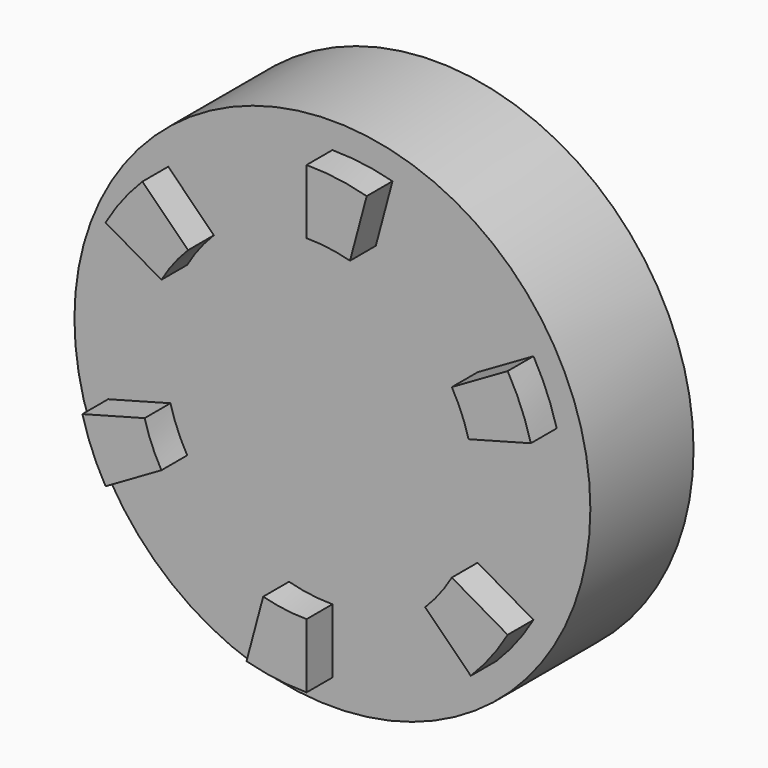
from build123d import *

# Parameters (mm, degrees)
F0_R     = 25.4
F1_DEPTH = 12.7
F2_DEPTH = 15.875


# Not quite as in the source:
# - a length typed as a fraction of an inch, garbled in the dataset ("3 / 203.2 mm" for 3/8 in), is restored
# - a feature names something its author has since deleted; it is built from what else it names


with BuildPart() as f1:
    # F0 (on Front) → F1 (new body)
    with BuildSketch(Plane.XZ):
        Circle(F0_R)
        with BuildLine():
            Line((0, -16.51), (0, -22.86))
            ThreePointArc((0, -22.86), (-2.9838287542, -22.664429531), (-5.916603371, -22.081064389))
            Line((-5.916603371, -22.081064389), (-4.2731024346, -15.947435392))
            ThreePointArc((-4.2731024346, -15.947435392), (-2.1549874336, -16.3687546613), (0, -16.51))
        make_face(mode=Mode.SUBTRACT)
        with BuildLine():
            Line((-14.2980794165, -8.255), (-19.7973407305, -11.43))
            ThreePointArc((-19.7973407305, -11.43), (-21.1198861132, -8.7481432639), (-22.081064389, -5.916603371))
            Line((-22.081064389, -5.916603371), (-15.947435392, -4.2731024346))
            ThreePointArc((-15.947435392, -4.2731024346), (-15.2532510818, -6.3181034683), (-14.2980794165, -8.255))
        make_face(mode=Mode.SUBTRACT)
        with BuildLine():
            Line((14.2980794165, -8.255), (19.7973407305, -11.43))
            ThreePointArc((19.7973407305, -11.43), (18.1360573591, -13.9162862671), (16.1644610179, -16.1644610179))
            Line((16.1644610179, -16.1644610179), (11.6743329574, -11.6743329574))
            ThreePointArc((11.6743329574, -11.6743329574), (13.0982636482, -10.0506511929), (14.2980794165, -8.255))
        make_face(mode=Mode.SUBTRACT)
        with BuildLine():
            Line((-14.2980794165, 8.255), (-19.7973407305, 11.43))
            ThreePointArc((-19.7973407305, 11.43), (-18.1360573591, 13.9162862671), (-16.1644610179, 16.1644610179))
            Line((-16.1644610179, 16.1644610179), (-11.6743329574, 11.6743329574))
            ThreePointArc((-11.6743329574, 11.6743329574), (-13.0982636482, 10.0506511929), (-14.2980794165, 8.255))
        make_face(mode=Mode.SUBTRACT)
        with BuildLine():
            Line((14.2980794165, 8.255), (19.7973407305, 11.43))
            ThreePointArc((19.7973407305, 11.43), (21.1198861132, 8.7481432639), (22.081064389, 5.916603371))
            Line((22.081064389, 5.916603371), (15.947435392, 4.2731024346))
            ThreePointArc((15.947435392, 4.2731024346), (15.2532510818, 6.3181034683), (14.2980794165, 8.255))
        make_face(mode=Mode.SUBTRACT)
        with BuildLine():
            Line((0, 16.51), (0, 22.86))
            ThreePointArc((0, 22.86), (2.9838287542, 22.664429531), (5.916603371, 22.081064389))
            Line((5.916603371, 22.081064389), (4.2731024346, 15.947435392))
            ThreePointArc((4.2731024346, 15.947435392), (2.1549874336, 16.3687546613), (0, 16.51))
        make_face(mode=Mode.SUBTRACT)
        with BuildLine():
            ThreePointArc((5.916603371, 22.081064389), (2.9838287542, 22.664429531), (0, 22.86))
            Line((0, 22.86), (0, 16.51))
            ThreePointArc((0, 16.51), (2.1549874336, 16.3687546613), (4.2731024346, 15.947435392))
            Line((4.2731024346, 15.947435392), (5.916603371, 22.081064389))
        make_face()
        with BuildLine():
            ThreePointArc((-16.1644610179, 16.1644610179), (-18.1360573591, 13.9162862671), (-19.7973407305, 11.43))
            Line((-19.7973407305, 11.43), (-14.2980794165, 8.255))
            ThreePointArc((-14.2980794165, 8.255), (-13.0982636482, 10.0506511929), (-11.6743329574, 11.6743329574))
            Line((-11.6743329574, 11.6743329574), (-16.1644610179, 16.1644610179))
        make_face()
        with BuildLine():
            ThreePointArc((-22.081064389, -5.916603371), (-21.1198861132, -8.7481432639), (-19.7973407305, -11.43))
            Line((-19.7973407305, -11.43), (-14.2980794165, -8.255))
            ThreePointArc((-14.2980794165, -8.255), (-15.2532510818, -6.3181034683), (-15.947435392, -4.2731024346))
            Line((-15.947435392, -4.2731024346), (-22.081064389, -5.916603371))
        make_face()
        with BuildLine():
            ThreePointArc((16.1644610179, -16.1644610179), (18.1360573591, -13.9162862671), (19.7973407305, -11.43))
            Line((19.7973407305, -11.43), (14.2980794165, -8.255))
            ThreePointArc((14.2980794165, -8.255), (13.0982636482, -10.0506511929), (11.6743329574, -11.6743329574))
            Line((11.6743329574, -11.6743329574), (16.1644610179, -16.1644610179))
        make_face()
        with BuildLine():
            ThreePointArc((22.081064389, 5.916603371), (21.1198861132, 8.7481432639), (19.7973407305, 11.43))
            Line((19.7973407305, 11.43), (14.2980794165, 8.255))
            ThreePointArc((14.2980794165, 8.255), (15.2532510818, 6.3181034683), (15.947435392, 4.2731024346))
            Line((15.947435392, 4.2731024346), (22.081064389, 5.916603371))
        make_face()
        with BuildLine():
            ThreePointArc((-5.916603371, -22.081064389), (-2.9838287542, -22.664429531), (0, -22.86))
            Line((0, -22.86), (0, -16.51))
            ThreePointArc((0, -16.51), (-2.1549874336, -16.3687546613), (-4.2731024346, -15.947435392))
            Line((-4.2731024346, -15.947435392), (-5.916603371, -22.081064389))
        make_face()
    extrude(amount=F1_DEPTH)

    # F0 (on Front) → F2 (join)
    with BuildSketch(Plane.XZ):
        with BuildLine():
            ThreePointArc((22.081064389, 5.916603371), (21.1198861132, 8.7481432639), (19.7973407305, 11.43))
            Line((19.7973407305, 11.43), (14.2980794165, 8.255))
            ThreePointArc((14.2980794165, 8.255), (15.2532510818, 6.3181034683), (15.947435392, 4.2731024346))
            Line((15.947435392, 4.2731024346), (22.081064389, 5.916603371))
        make_face()
        with BuildLine():
            ThreePointArc((16.1644610179, -16.1644610179), (18.1360573591, -13.9162862671), (19.7973407305, -11.43))
            Line((19.7973407305, -11.43), (14.2980794165, -8.255))
            ThreePointArc((14.2980794165, -8.255), (13.0982636482, -10.0506511929), (11.6743329574, -11.6743329574))
            Line((11.6743329574, -11.6743329574), (16.1644610179, -16.1644610179))
        make_face()
        with BuildLine():
            ThreePointArc((-5.916603371, -22.081064389), (-2.9838287542, -22.664429531), (0, -22.86))
            Line((0, -22.86), (0, -16.51))
            ThreePointArc((0, -16.51), (-2.1549874336, -16.3687546613), (-4.2731024346, -15.947435392))
            Line((-4.2731024346, -15.947435392), (-5.916603371, -22.081064389))
        make_face()
        with BuildLine():
            ThreePointArc((-16.1644610179, 16.1644610179), (-18.1360573591, 13.9162862671), (-19.7973407305, 11.43))
            Line((-19.7973407305, 11.43), (-14.2980794165, 8.255))
            ThreePointArc((-14.2980794165, 8.255), (-13.0982636482, 10.0506511929), (-11.6743329574, 11.6743329574))
            Line((-11.6743329574, 11.6743329574), (-16.1644610179, 16.1644610179))
        make_face()
        with BuildLine():
            ThreePointArc((5.916603371, 22.081064389), (2.9838287542, 22.664429531), (0, 22.86))
            Line((0, 22.86), (0, 16.51))
            ThreePointArc((0, 16.51), (2.1549874336, 16.3687546613), (4.2731024346, 15.947435392))
            Line((4.2731024346, 15.947435392), (5.916603371, 22.081064389))
        make_face()
        with BuildLine():
            ThreePointArc((-22.081064389, -5.916603371), (-21.1198861132, -8.7481432639), (-19.7973407305, -11.43))
            Line((-19.7973407305, -11.43), (-14.2980794165, -8.255))
            ThreePointArc((-14.2980794165, -8.255), (-15.2532510818, -6.3181034683), (-15.947435392, -4.2731024346))
            Line((-15.947435392, -4.2731024346), (-22.081064389, -5.916603371))
        make_face()
    extrude(amount=F2_DEPTH)


solid = f1.part
